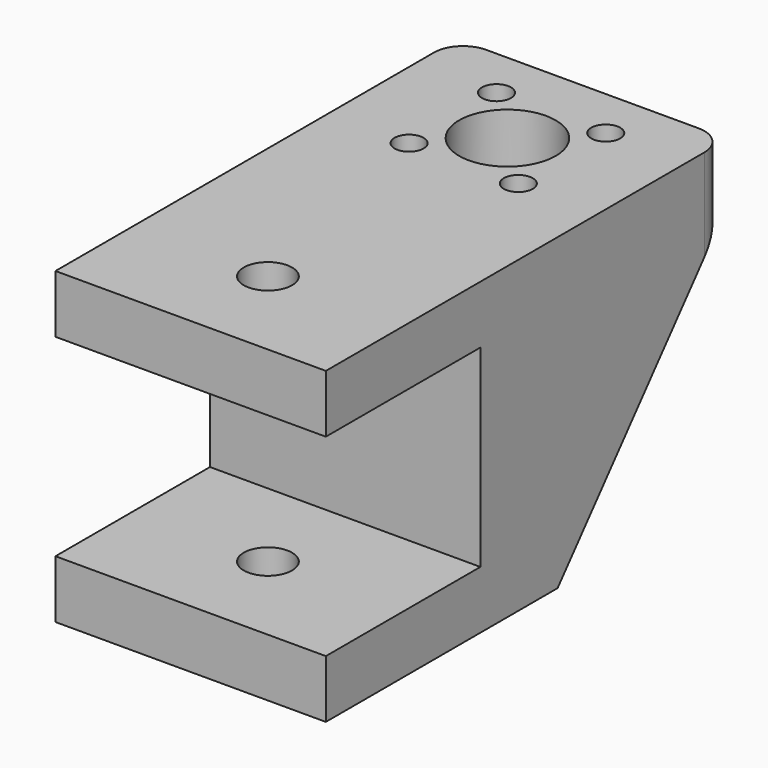
from build123d import *

# Parameters (mm, degrees)
F0_W          = 22
F0_H          = 22
F0_R          = 1.5
F0_R_2        = 5
F1_DEPTH      = 6
F2_W          = 22
F2_H          = 32
F3_DEPTH      = 10
F4_W          = 22
F4_H          = 6
F5_DEPTH      = 20
F6_R          = 2.5
F7_DEPTH      = 32.001
F9_DEPTH      = 3
F11_DEPTH     = 3
F12_T1_DEPTH  = 21
F12_T6_DEPTH  = 5.7473088859
F12_S7_R      = 3
F12_T8_DEPTH  = 5
F12_T12_DEPTH = 5.7473088859
F12_S13_R     = 3
F12_T14_DEPTH = 5


# Not quite as in the source:
# - a fillet or chamfer that OpenCascade refuses, or shapes differently, is made with other operations: its cross-section is extruded or revolved along the edge and cut away or added
# - a feature of the source that left no trace in its solid (it failed there, or was rolled back) is left out


with BuildPart() as f1:
    # F0 (on Top) → F1 (new body)
    with BuildSketch(Plane.XY):
        with Locations((-50.6666042507, 16.1375404)):
            Rectangle(F0_W, F0_H)
        with Locations((-56.3234585002, 10.4806861505)):
            Circle(F0_R, mode=Mode.SUBTRACT)
        with Locations((-45.0097500012, 10.4806861505)):
            Circle(F0_R, mode=Mode.SUBTRACT)
        with Locations((-50.6666042507, 16.1375404)):
            Circle(F0_R_2, mode=Mode.SUBTRACT)
        with Locations((-56.3234585002, 21.7943946495)):
            Circle(F0_R, mode=Mode.SUBTRACT)
        with Locations((-45.0097500012, 21.7943946495)):
            Circle(F0_R, mode=Mode.SUBTRACT)
    extrude(amount=F1_DEPTH)

    # F2 (on face) → F3 (join)
    with BuildSketch(Plane.XZ.offset(-5.1375404)):
        with Locations((-50.6666042507, -10)):
            Rectangle(F2_W, F2_H)
    extrude(amount=F3_DEPTH)

    # F4 (on face) → F5 (join)
    with BuildSketch(Plane.XZ.offset(4.8624596)):
        with Locations((-50.6666042507, 3)):
            Rectangle(F4_W, F4_H)
        with Locations((-50.6666042507, -23)):
            Rectangle(F4_W, F4_H)
    extrude(amount=F5_DEPTH)

    # F6 (on face) → F7 (cut, through all)
    with BuildSketch(Plane.XY.offset(6)):
        with Locations((-50.6666042507, -14.8624596)):
            Circle(F6_R)
    extrude(amount=-F7_DEPTH, mode=Mode.SUBTRACT)

    # F8 (on face) → F9 (join)
    with BuildSketch(Plane(origin=(-61.6666042507, 0, 0), x_dir=(0, -1, 0), z_dir=(-1, 0, 0))):
        Polygon((-27.1375404, 0), (-5.1375404, -26), (-5.1375404, 0), align=None)
        Polygon((-5.1375404, 0), (-5.1375404, -26), (24.8624596, -26), (24.8624596, -20), (4.8624596, -20), (4.8624596, 0), (24.8624596, 0), (24.8624596, 6), (-27.1375404, 6), (-27.1375404, 0), align=None)
    extrude(amount=F9_DEPTH)

    # F10 (on face) → F11 (join)
    with BuildSketch(Plane.YZ.offset(-39.6666042507)):
        Polygon((5.1375404, 0), (5.1375404, -26), (27.1375404, 0), align=None)
        Polygon((-24.8624596, -26), (5.1375404, -26), (5.1375404, 0), (27.1375404, 0), (27.1375404, 6), (-24.8624596, 6), (-24.8624596, 0), (-4.8624596, 0), (-4.8624596, -20), (-24.8624596, -20), align=None)
    extrude(amount=F11_DEPTH)

    # F12: fillet of radius 3 on 4 edges, made by hand

    # F12_s2 → F12_t1 (cut)
    with BuildSketch(Plane.XY.offset(-7.5)):
        with BuildLine():
            ThreePointArc((-61.6666042507, 27.1375404), (-63.7879245942, 26.2588607436), (-64.6666042507, 24.1375404))
            Line((-64.6666042507, 24.1375404), (-64.6666042507, 27.1375404))
            Line((-64.6666042507, 27.1375404), (-61.6666042507, 27.1375404))
        make_face()
        with BuildLine():
            ThreePointArc((-39.6666042507, 27.1375404), (-37.5452839071, 26.2588607436), (-36.6666042507, 24.1375404))
            Line((-36.6666042507, 24.1375404), (-36.6666042507, 27.1375404))
            Line((-36.6666042507, 27.1375404), (-39.6666042507, 27.1375404))
        make_face()
    extrude(amount=F12_T1_DEPTH, mode=Mode.SUBTRACT)


with BuildPart() as f12_tool4:
    # F12_s5 → F12_t6 (new body)
    with BuildSketch(Plane.YZ.offset(-61.6666042507)):
        with BuildLine():
            ThreePointArc((27.1375404, 1.0989235543), (26.9544958992, 0.0670506378), (26.4276992561, -0.8389031701))
            Line((26.4276992561, -0.8389031701), (27.1375404, 0))
            Line((27.1375404, 0), (27.1375404, 1.0989235543))
        make_face()
    extrude(amount=-F12_T6_DEPTH)

    # F12_s7 → F12_t8 (cut, symmetric)
    with BuildSketch(Plane.XY.offset(0.1)):
        with Locations((-61.6666042507, 24.1375404)):
            Circle(F12_S7_R)
    extrude(amount=F12_T8_DEPTH, both=True, mode=Mode.SUBTRACT)


with BuildPart() as f1_1:
    add(f1.part)

    # F12_t3: cut F12_tool4
    add(f12_tool4.part, mode=Mode.SUBTRACT)


with BuildPart() as f12_tool10:
    # F12_s11 → F12_t12 (new body)
    with BuildSketch(Plane.YZ.offset(-39.6666042507)):
        with BuildLine():
            ThreePointArc((27.1375404, 1.0989235543), (26.9544958992, 0.0670506378), (26.4276992561, -0.8389031701))
            Line((26.4276992561, -0.8389031701), (27.1375404, 0))
            Line((27.1375404, 0), (27.1375404, 1.0989235543))
        make_face()
    extrude(amount=F12_T12_DEPTH)

    # F12_s13 → F12_t14 (cut, symmetric)
    with BuildSketch(Plane.XY.offset(0.1)):
        with Locations((-39.6666042507, 24.1375404)):
            Circle(F12_S13_R)
    extrude(amount=F12_T14_DEPTH, both=True, mode=Mode.SUBTRACT)


with BuildPart() as f1_2:
    add(f1_1.part)

    # F12_t9: cut F12_tool10
    add(f12_tool10.part, mode=Mode.SUBTRACT)


solid = f1_2.part
